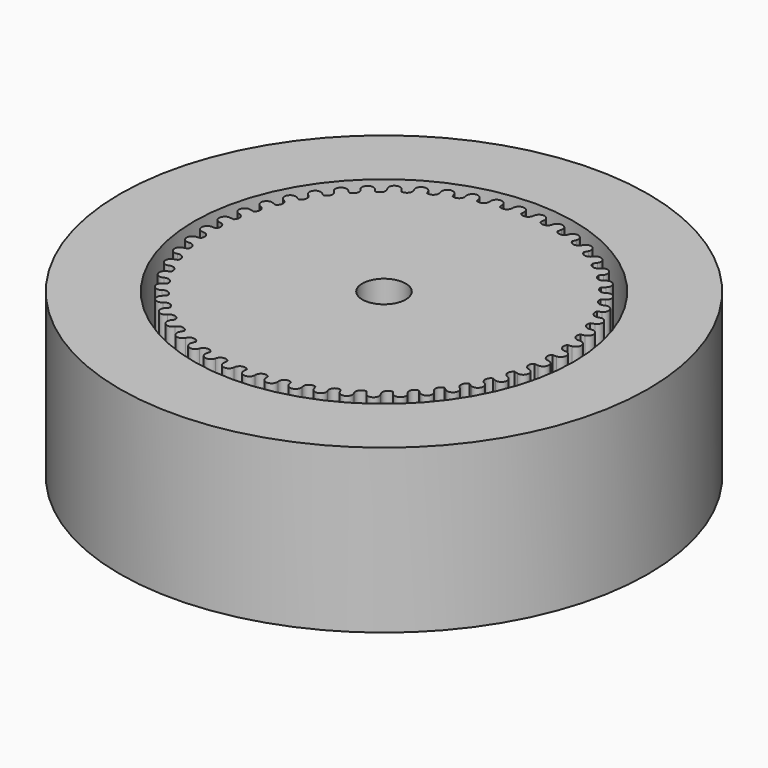
from build123d import *

# Parameters (mm, degrees)
F0_R            = 48.6627366637
F5_DEPTH        = 30
F1_R            = 35.0000150506
F6_DEPTH        = 30.001
F6_DEPTH_BACK   = 156
F2_R            = 30.9265383117
F7_DEPTH        = 30
F3_R            = 4
F8_DEPTH        = 156
F8_DEPTH_BACK   = 30.001
F9_DEPTH        = 30
F9_COPIES_COUNT = 52


# Not quite as in the source:
# - an extrude ends at something that could not be found from the text; its depth is read off the source's solid
# - a pattern or mirror of a feature is missing from the dataset's text; its kind, count and spacing are read off the source's solid


with BuildPart() as f5:
    # F0 (on Top) → F5 (new body)
    with BuildSketch(Plane.XY):
        Circle(F0_R)
    extrude(amount=F5_DEPTH)

    # F1 (on Top) → F6 (cut, two sides)
    with BuildSketch(Plane.XY) as f6_sk:
        Circle(F1_R)
    extrude(amount=F6_DEPTH, mode=Mode.SUBTRACT)
    extrude(f6_sk.sketch, amount=-F6_DEPTH_BACK, mode=Mode.SUBTRACT)


with BuildPart() as f7:
    # F2 (on Top) → F7 (new body)
    with BuildSketch(Plane.XY):
        Circle(F2_R)
    extrude(amount=F7_DEPTH)

    # F3 (on Top) → F8 (cut, two sides)
    with BuildSketch(Plane.XY) as f8_sk:
        Circle(F3_R)
    extrude(amount=-F8_DEPTH, mode=Mode.SUBTRACT)
    extrude(f8_sk.sketch, amount=F8_DEPTH_BACK, mode=Mode.SUBTRACT)

    # F4 (on Top) → F9 (join)
    with BuildSketch(Plane.XY):
        with BuildLine():
            ThreePointArc((2.0724304561, 31.9035298274), (1.0031356089, 30.9176046092), (0, 31.9707707672))
            Line((0, 31.9707707672), (0, 24.8469758109))
            Line((0, 24.8469758109), (3.2417628131, 24.8469758109))
            Line((3.2417628131, 24.8469758109), (4.1361434388, 31.7020898507))
            ThreePointArc((4.1361434388, 31.7020898507), (3.2066537045, 32.8515371516), (2.0724304561, 31.9035298274))
        make_face()
    f9 = extrude(amount=F9_DEPTH)

    # F9_copies: F9 ×52 about axis
    f9_copies_axis = Axis((0, 0, 0), (0, 0, 1))
    for i in range(1, F9_COPIES_COUNT):
        add(f9.rotate(f9_copies_axis, i * 360 / F9_COPIES_COUNT))


solid = Compound([f5.part, f7.part])
